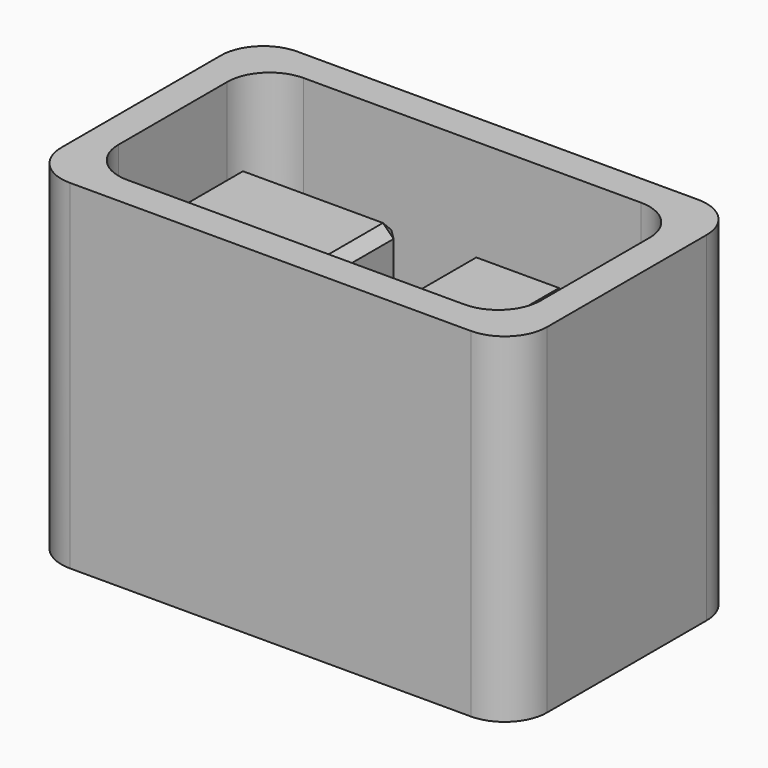
from build123d import *

# Parameters (mm, degrees)
F0_W     = 22.9
F0_H     = 13.4
F1_DEPTH = 2
F2_W     = 22.9
F2_H     = 13.4
F2_W_2   = 19.9
F2_H_2   = 10.4
F3_DEPTH = 14
F4_W     = 15.9
F4_H     = 6.4
F5_DEPTH = 12
F6_W     = 7.6
F6_H     = 1.698620432
F6_W_2   = 4.9
F7_DEPTH = 8
F8_W     = 3.4
F8_H     = 6.4
F9_DEPTH = 4
F10_SIZE = 0.5
F11_R    = 2


with BuildPart() as f1:
    # F0 (on Top) → F1 (new body)
    with BuildSketch(Plane.XY):
        Rectangle(F0_W, F0_H)
    extrude(amount=F1_DEPTH)

    # F2 (on face) → F3 (join)
    with BuildSketch(Plane.XY.offset(2)):
        Rectangle(F2_W, F2_H)
        Rectangle(F2_W_2, F2_H_2, mode=Mode.SUBTRACT)
    extrude(amount=F3_DEPTH)

    # F4 (on face) → F5 (join)
    with BuildSketch(Plane.XY.offset(2)):
        Rectangle(F4_W, F4_H)
    extrude(amount=F5_DEPTH)

    # F6 (on face) → F7 (cut)
    with BuildSketch(Plane.XY.offset(14)):
        with Locations((-4.15, 2.350689784)):
            Rectangle(F6_W, F6_H)
        Polygon((-0.35, 3.2), (-0.35, 1.501379568), (-0.35, -3.2), (3.05, -3.2), (3.05, 1.501379568), (3.05, 3.2), align=None)
        with Locations((5.5, 2.350689784)):
            Rectangle(F6_W_2, F6_H)
    extrude(amount=-F7_DEPTH, mode=Mode.SUBTRACT)

    # F8 (on face) → F9 (cut)
    with BuildSketch(Plane.XY.offset(6)):
        with Locations((1.35, 0)):
            Rectangle(F8_W, F8_H)
    extrude(amount=-F9_DEPTH, mode=Mode.SUBTRACT)

    # F10
    f10_edges = [f1.edges().sort_by_distance(p)[0] for p in [
        (-4.15, 1.50138, 14),
        (-0.35, -0.84931, 14),
        (-4.15, -3.2, 14),
        (-7.95, -0.84931, 14),
        (-7.95, 1.50138, 10),
        (-0.35, 1.50138, 10),
        (-0.35, -3.2, 8),
        (3.05, -3.2, 8),
        (7.95, -0.84931, 14),
        (5.5, -3.2, 14),
        (3.05, -0.84931, 14),
        (5.5, 1.50138, 14),
        (7.95, 1.50138, 10),
        (3.05, 1.50138, 10),
        (3.05, 3.2, 4),
        (7.95, 3.2, 4),
        (7.95, -3.2, 8),
        (-0.35, 3.2, 4),
        (-7.95, 3.2, 4),
        (-7.95, -3.2, 8),
    ]]
    chamfer(f10_edges, length=F10_SIZE)

    # F11
    f11_edges = [f1.edges().sort_by_distance(p)[0] for p in [
        (9.95, -5.2, 9),
        (9.95, 5.2, 9),
        (-9.95, 5.2, 9),
        (-9.95, -5.2, 9),
        (11.45, -6.7, 8),
        (11.45, 6.7, 8),
        (-11.45, 6.7, 8),
        (-11.45, -6.7, 8),
    ]]
    fillet(f11_edges, radius=F11_R)


solid = f1.part
